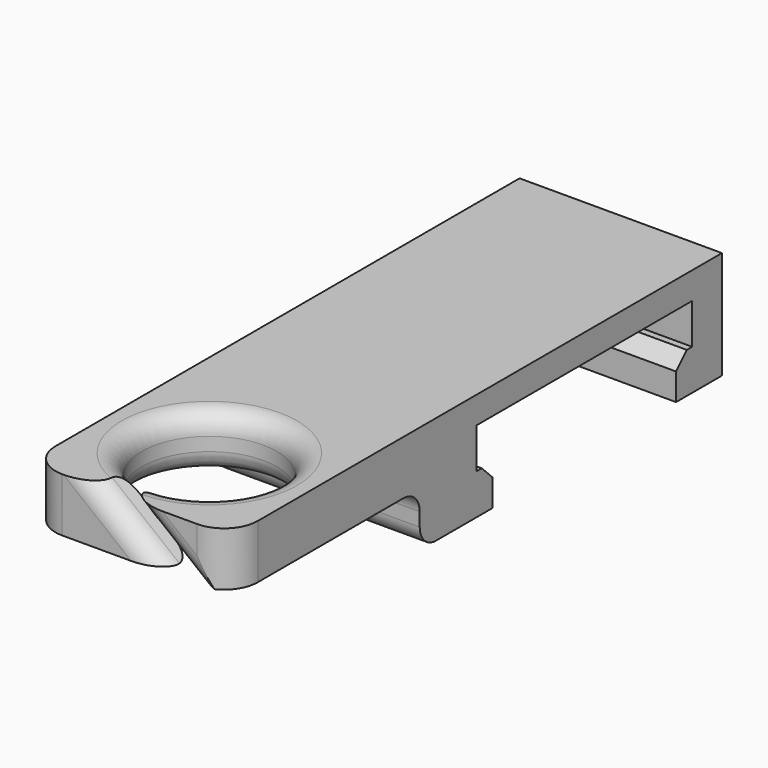
from build123d import *

# Parameters (mm, degrees)
F0_W          = 30
F0_H          = 56
F1_DEPTH      = 15
F1_DEPTH_BACK = 1
F2_START      = 7
F0_R          = 10
F2_DEPTH      = 8
F3_R          = 3
F4_R          = 3
F6_DEPTH      = 8
F7_T1_DEPTH   = 27.8062484749
F7_T3_DEPTH   = 27.8062484749
F9_DEPTH      = 30
F10_SIZE      = 2


# Not quite as in the source:
# - a fillet or chamfer that OpenCascade refuses, or shapes differently, is made with other operations: its cross-section is extruded or revolved along the edge and cut away or added


with BuildPart() as f1:
    # F0 (on Top) → F1 (new body, two sides)
    with BuildSketch(Plane.XY) as f1_sk:
        with Locations((0, 17.5)):
            Rectangle(F0_W, F0_H)
    extrude(amount=F1_DEPTH)
    extrude(f1_sk.sketch, amount=-F1_DEPTH_BACK)

    # F0 (on Top) → F2 (join)
    with BuildSketch(Plane.XY.offset(F2_START)):
        with BuildLine():
            Line((15, -40.5), (15, -10.5))
            Line((15, -10.5), (-15, -10.5))
            Line((-15, -10.5), (-15, -40.5))
            ThreePointArc((-15, -40.5), (-13.5355339059, -44.0355339059), (-10, -45.5))
            Line((-10, -45.5), (10, -45.5))
            ThreePointArc((10, -45.5), (13.5355339059, -44.0355339059), (15, -40.5))
        make_face()
        with Locations((0, -30.7424795181)):
            Circle(F0_R, mode=Mode.SUBTRACT)
    extrude(amount=F2_DEPTH)

    # F3
    f3_edges = [f1.edges().sort_by_distance(p)[0] for p in [
        (0, -10.5, 7),
        (0, -10.5, -1),
    ]]
    fillet(f3_edges, radius=F3_R)

    # F4
    f4_edges = [f1.edges().sort_by_distance(p)[0] for p in [
        (-10, -30.74248, 15),
        (-10, -30.74248, 7),
    ]]
    fillet(f4_edges, radius=F4_R)

    # F5 (on face) → F6 (cut)
    with BuildSketch(Plane.XZ.offset(45.5)):
        Polygon((10, 7), (0, 15), (-5, 15), (5, 7), align=None)
    extrude(amount=-F6_DEPTH, mode=Mode.SUBTRACT)

    # F7: fillet of radius 3 on 2 edges, made by hand

    # F7_s2 → F7_t1 (cut)
    with BuildSketch(Plane(origin=(-16.2223697294, 0, 12.9778957835), x_dir=(0, 1, 0), z_dir=(0.7808688094, 0, -0.6246950476))):
        with BuildLine():
            ThreePointArc((-45.5, 5.5895569039), (-44.6213203436, 7.7108772474), (-42.5, 8.5895569039))
            Line((-42.5, 8.5895569039), (-45.5, 8.5895569039))
            Line((-45.5, 8.5895569039), (-45.5, 5.5895569039))
        make_face()
    extrude(amount=F7_T1_DEPTH, mode=Mode.SUBTRACT)

    # F7_s4 → F7_t3 (cut)
    with BuildSketch(Plane(origin=(8.5394429001, 0, -6.8315543201), x_dir=(0, 1, 0), z_dir=(-0.7808688094, 0, 0.6246950476))):
        with BuildLine():
            ThreePointArc((-45.5, -14.7130321416), (-44.6213203436, -12.5917117981), (-42.5, -11.7130321416))
            Line((-42.5, -11.7130321416), (-45.5, -11.7130321416))
            Line((-45.5, -11.7130321416), (-45.5, -14.7130321416))
        make_face()
    extrude(amount=F7_T3_DEPTH, mode=Mode.SUBTRACT)

    # F8 (on face) → F9 (cut, through all)
    with BuildSketch(Plane(origin=(-15, 0, 0), x_dir=(0, -1, 0), z_dir=(-1, 0, 0))):
        Polygon((0, 5), (0, 11), (-40, 11), (-40, 10), (-40, 5), (-37, 5), (-37, -1), (-3, -1), (-3, 5), align=None)
    extrude(amount=-F9_DEPTH, mode=Mode.SUBTRACT)

    # F10
    f10_edges = [f1.edges().sort_by_distance(p)[0] for p in [
        (0, 37, 5),
        (0, 3, 5),
    ]]
    chamfer(f10_edges, length=F10_SIZE)


solid = f1.part
